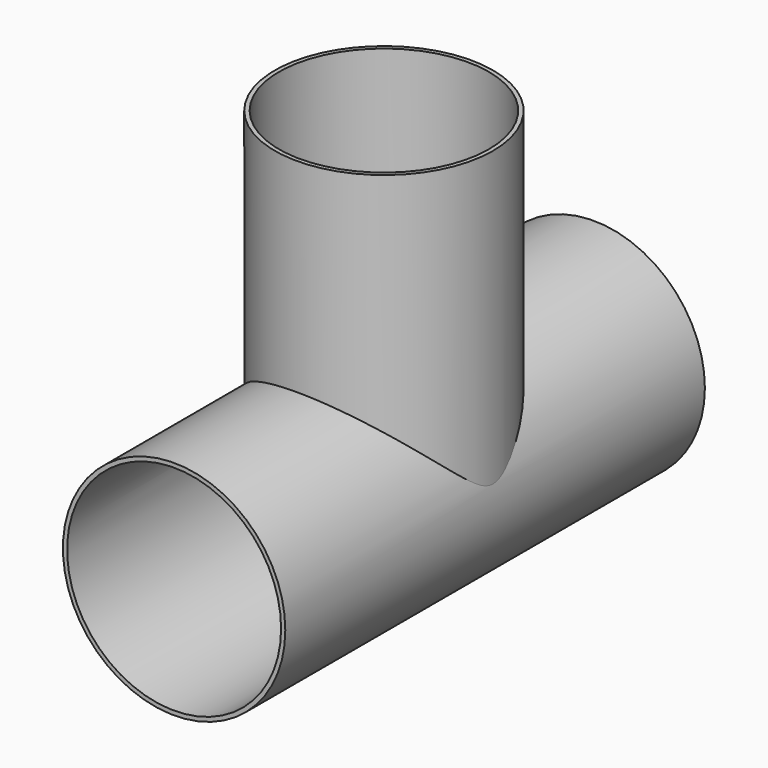
from build123d import *

# Parameters (mm, degrees)
F0_R     = 53
F0_R_2   = 51
F1_DEPTH = 250
F3_R     = 52
F3_R_2   = 50
F4_REACH = 350.0792104868
F5_R     = 50
F6_REACH = 344.4223563373


with BuildPart() as f1:
    # F0 (on Front) → F1 (new body)
    with BuildSketch(Plane.XZ):
        Circle(F0_R)
        Circle(F0_R_2, mode=Mode.SUBTRACT)
    extrude(amount=-F1_DEPTH)

    f4_end = f1.faces().sort_by_distance((-53, 125, 0))[0]
    # F3 (on offset) → F4 (join, up to a face of the model that its end follows)
    with BuildSketch(Plane.XY.offset(150)):
        with Locations((0, 125.0192821026)):
            Circle(F3_R)
        with Locations((0, 125.0192821026)):
            Circle(F3_R_2, mode=Mode.SUBTRACT)
    f4_long = extrude(amount=-F4_REACH, mode=Mode.PRIVATE)
    add(split(f4_long, bisect_by=f4_end, keep=Keep.ALL, mode=Mode.PRIVATE).solids().sort_by_distance((-50.5292178951, 125.0192821026, 150))[0])

    f6_end = f1.faces().sort_by_distance((-51, 125, 0))[0]
    # F5 (on offset) → F6 (cut, up to a face of the model that its end follows)
    with BuildSketch(Plane.XY.offset(150)):
        with Locations((0, 125.0192821026)):
            Circle(F5_R)
    f6_long = extrude(amount=-F6_REACH, mode=Mode.PRIVATE)
    add(split(f6_long, bisect_by=f6_end, keep=Keep.ALL, mode=Mode.PRIVATE).solids().sort_by_distance((0, 125.0192821026, 150))[0], mode=Mode.SUBTRACT)


solid = f1.part
